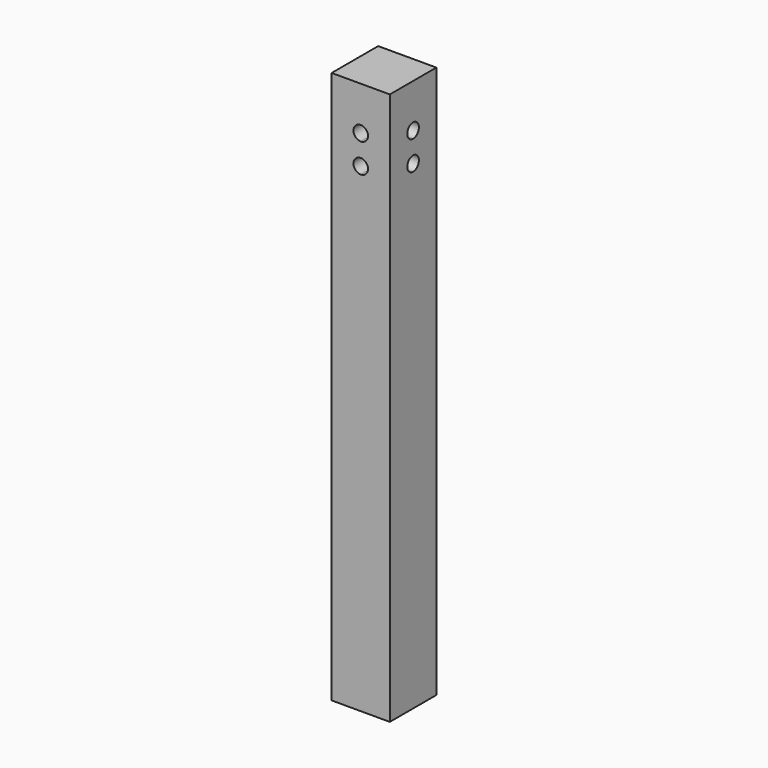
from build123d import *

# Parameters (mm, degrees)
F0_W     = 101.6
F0_H     = 965.2
F1_DEPTH = 101.6
F3_DEPTH = 101.601
F5_DEPTH = 101.601


with BuildPart() as f1:
    # F0 (on Front) → F1 (new body)
    with BuildSketch(Plane.XZ):
        with Locations((50.8, 482.6)):
            Rectangle(F0_W, F0_H)
    extrude(amount=F1_DEPTH)

    # F2 (on face) → F3 (cut, through all)
    with BuildSketch(Plane.XZ.offset(101.6)):
        with BuildLine():
            ThreePointArc((63.5, 889), (59.7802561211, 897.9802561211), (50.8, 901.7))
            Line((50.8, 901.7), (50.8, 876.3))
            ThreePointArc((50.8, 876.3), (59.7802561211, 880.0197438789), (63.5, 889))
        make_face()
        with BuildLine():
            ThreePointArc((63.5, 838.2), (59.7802561211, 847.1802561211), (50.8, 850.9))
            Line((50.8, 850.9), (50.8, 825.5))
            ThreePointArc((50.8, 825.5), (59.7802561211, 829.2197438789), (63.5, 838.2))
        make_face()
        with BuildLine():
            Line((50.8, 825.5), (50.8, 850.9))
            ThreePointArc((50.8, 850.9), (38.1, 838.2), (50.8, 825.5))
        make_face()
        with BuildLine():
            Line((50.8, 876.3), (50.8, 901.7))
            ThreePointArc((50.8, 901.7), (38.1, 889), (50.8, 876.3))
        make_face()
    extrude(amount=-F3_DEPTH, mode=Mode.SUBTRACT)

    # F4 (on face) → F5 (cut, through all)
    with BuildSketch(Plane(origin=(0, 0, 0), x_dir=(0, -1, 0), z_dir=(-1, 0, 0))):
        with BuildLine():
            ThreePointArc((63.5, 889), (59.7802561211, 897.9802561211), (50.8, 901.7))
            Line((50.8, 901.7), (50.8, 876.3))
            ThreePointArc((50.8, 876.3), (59.7802561211, 880.0197438789), (63.5, 889))
        make_face()
        with BuildLine():
            ThreePointArc((63.5, 838.2), (59.7802561211, 847.1802561211), (50.8, 850.9))
            Line((50.8, 850.9), (50.8, 825.5))
            ThreePointArc((50.8, 825.5), (59.7802561211, 829.2197438789), (63.5, 838.2))
        make_face()
        with BuildLine():
            Line((50.8, 825.5), (50.8, 850.9))
            ThreePointArc((50.8, 850.9), (38.1, 838.2), (50.8, 825.5))
        make_face()
        with BuildLine():
            Line((50.8, 876.3), (50.8, 901.7))
            ThreePointArc((50.8, 901.7), (38.1, 889), (50.8, 876.3))
        make_face()
    extrude(amount=-F5_DEPTH, mode=Mode.SUBTRACT)


solid = f1.part
